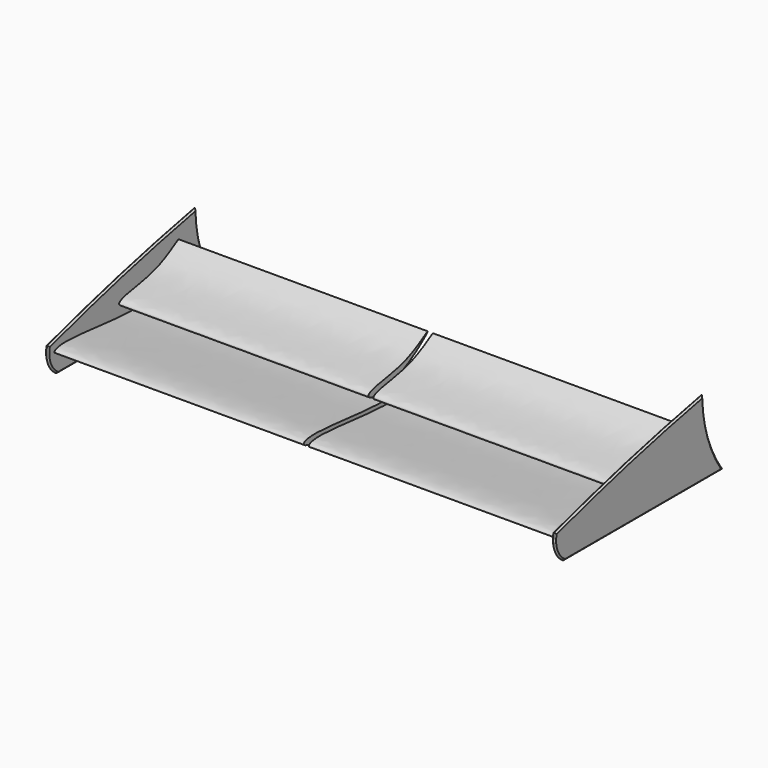
from build123d import *

# Parameters (mm, degrees)
F2_DEPTH = 772
F4_DEPTH = 10
F5_SIZE  = 4.99999


# Not quite as in the source:
# - a fillet or chamfer is up to 0.001 mm smaller than in the source, because OpenCascade refuses the exact size


with BuildPart() as f2:
    # F1 (on offset) → F2 (new body)
    with BuildSketch(Plane.YZ.offset(780)):
        with BuildLine():
            add(Edge.make_bspline(
                [(-1744.877576828, 58.9434765279), (-1745.3802478559, 61.5366577599), (-1832.0368493958, 45.8225946383), (-2078.2755369764, 86.2614809539), (-2127.8559983427, 65.176742592), (-2081.002772978, 44.746449474), (-1828.8614657532, 25.1825377325), (-1744.3728278282, 56.3395754464), (-1744.877576828, 58.9434765279)],
                knots=[0, 0, 0, 0, 0.139792449, 0.4094320274, 0.4995044186, 0.5885009526, 0.8596296685, 1, 1, 1, 1], degree=3))
        make_face()
    extrude(amount=-F2_DEPTH)



with BuildPart() as f2b:
    # F1 (on offset) → F2, piece 2 (new body)
    with BuildSketch(Plane.YZ.offset(780)):
        with BuildLine():
            add(Edge.make_bspline(
                [(-1637.5484834412, 177.2178078336), (-1638.8543316655, 178.7057145257), (-1720.620327133, 118.8435706221), (-1845.0060490817, 113.6126241583), (-1875.2446737796, 93.082491228), (-1837.6845680548, 74.5660088647), (-1713.9329969259, 107.5802112125), (-1636.2257141975, 175.710621031), (-1637.5484834412, 177.2178078336)],
                knots=[0, 0, 0, 0, 0.1800131474, 0.4069173565, 0.4941344226, 0.5887229388, 0.8176542646, 1, 1, 1, 1], degree=3))
        make_face()
    extrude(amount=-F2_DEPTH)


with BuildPart() as f2_1:
    add(f2.part)

    add(f2b.part)  # F4 merges F2b
    # F3 (on face) → F4 (join)
    with BuildSketch(Plane.YZ.offset(780)):
        with BuildLine():
            ThreePointArc((-2140.186571362, 89.9610519409), (-2137.3994155737, 39.0730721669), (-2104.6786308289, 0))
            Line((-2104.6786308289, 0), (-1489.6786308289, 0))
            ThreePointArc((-1489.6786308289, 0), (-1546.1377249923, 110.9117451388), (-1567.3653118634, 233.5430383682))
            ThreePointArc((-1567.3653118634, 233.5430383682), (-1855.5631600625, 168.8821646693), (-2140.186571362, 89.9610519409))
        make_face()
        with BuildLine():
            add(Edge.make_bspline(
                [(-1744.877576828, 58.9434765279), (-1745.3802478559, 61.5366577599), (-1832.0368493958, 45.8225946383), (-2078.2755369764, 86.2614809539), (-2127.8559983427, 65.176742592), (-2081.002772978, 44.746449474), (-1828.8614657532, 25.1825377325), (-1744.3728278282, 56.3395754464), (-1744.877576828, 58.9434765279)],
                knots=[0, 0, 0, 0, 0.139792449, 0.4094320274, 0.4995044186, 0.5885009526, 0.8596296685, 1, 1, 1, 1], degree=3))
        make_face(mode=Mode.SUBTRACT)
        with BuildLine():
            add(Edge.make_bspline(
                [(-1744.877576828, 58.9434765279), (-1745.3802478559, 61.5366577599), (-1832.0368493958, 45.8225946383), (-2078.2755369764, 86.2614809539), (-2127.8559983427, 65.176742592), (-2081.002772978, 44.746449474), (-1828.8614657532, 25.1825377325), (-1744.3728278282, 56.3395754464), (-1744.877576828, 58.9434765279)],
                knots=[0, 0, 0, 0, 0.139792449, 0.4094320274, 0.4995044186, 0.5885009526, 0.8596296685, 1, 1, 1, 1], degree=3))
        make_face()
    extrude(amount=F4_DEPTH)

    # F5 (size 5 in the source; OpenCascade refuses exactly that, so slightly less here)
    f5_edges = [f2_1.edges().sort_by_distance(p)[0] for p in [
        (780, -1855.56316, 168.882165),
        (780, -1546.137725, 110.911745),
        (780, -2137.399416, 39.073072),
        (780, -1797.178631, 0),
        (790, -1855.56316, 168.882165),
        (790, -2137.399416, 39.073072),
        (790, -1797.178631, 0),
        (790, -1546.137725, 110.911745),
    ]]
    chamfer(f5_edges, length=F5_SIZE)


with BuildPart() as f6_1:
    # F6: instance of F2
    add(f2_1.part.mirror(Plane.YZ))


solid = Compound([f2_1.part, f6_1.part])
